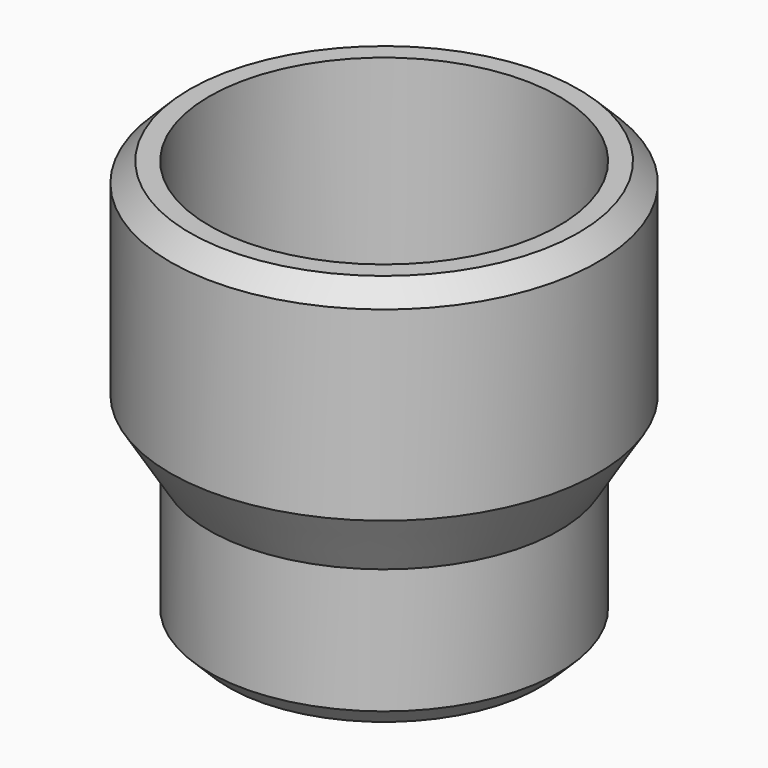
from build123d import *

# Parameters (mm, degrees)
F2_SIZE2 = 1
F2_SIZE  = 1
F3_SIZE2 = 0.99999
F3_SIZE  = 5.671272


# Not quite as in the source:
# - a fillet or chamfer is up to 0.001 mm smaller than in the source, because OpenCascade refuses the exact size


with BuildPart() as f1:
    # F0 (on Front) → F1 (revolve)
    with BuildSketch(Plane.XZ):
        Polygon((-9, 0), (-9, 10), (-11, 10), (-11, -0.5671153529), (-9, -3.8101770668), (-9, -11.2430617139), (-7, -11.2430617139), (-7, -3.2430617139), align=None)
    revolve(axis=Axis((0, 0, -1.2268370084), (0, 0, -1)))

    # F2
    f2_edges = [f1.edges().sort_by_distance(p)[0] for p in [
        (9, 0, -11.243062),
        (11, 0, 10),
    ]]
    chamfer(f2_edges, length=F2_SIZE, length2=F2_SIZE2)

    # F3 (size 5.6712818196 and 1 in the source; OpenCascade refuses exactly that, so slightly less here)
    f3_edges = [f1.edges().sort_by_distance(p)[0] for p in [
        (7, 0, -11.243062),
    ]]
    f3_side = f1.faces().sort_by_distance((7, 0, -7.243062))[0]
    chamfer(f3_edges, length=F3_SIZE, length2=F3_SIZE2, reference=f3_side)


solid = f1.part
